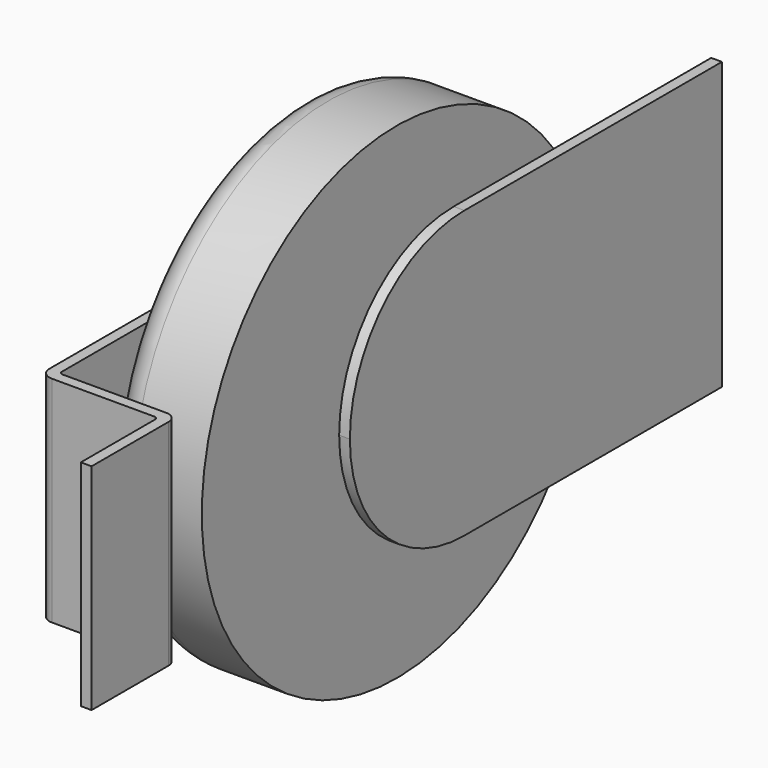
from build123d import *

# Parameters (mm, degrees)
F1_DEPTH      = 1.5
F1_DEPTH_BACK = 1.5
F4_DEPTH      = 2
F4_DEPTH_BACK = 2
F5_R          = 1.99999


# Not quite as in the source:
# - a fillet or chamfer is up to 0.001 mm smaller than in the source, because OpenCascade refuses the exact size


with BuildPart() as f1:
    # F0 (on Top) → F1 (new body, two sides)
    with BuildSketch(Plane.XY) as f1_sk:
        with BuildLine():
            Line((0.15, 1.5), (0, 1.5))
            Line((0, 1.5), (0, 0))
            Line((0, 0), (0, -4))
            ThreePointArc((0, -4), (0.0487994019, -4.1178121778), (0.1666115796, -4.1666115796))
            Line((0.1666115796, -4.1666115796), (1.6031347549, -4.1666115796))
            ThreePointArc((1.6031347549, -4.1666115796), (1.6362734875, -4.1803380921), (1.65, -4.2134768248))
            Line((1.65, -4.2134768248), (1.65, -5.5134768248))
            Line((1.65, -5.5134768248), (1.8, -5.5134768248))
            Line((1.8, -5.5134768248), (1.8, -4.1666115796))
            ThreePointArc((1.8, -4.1666115796), (1.7560660172, -4.0605455625), (1.65, -4.0166115796))
            Line((1.65, -4.0166115796), (0.1968652451, -4.0166115796))
            ThreePointArc((0.1968652451, -4.0166115796), (0.1637265125, -4.0028850671), (0.15, -3.9697463345))
            Line((0.15, -3.9697463345), (0.15, 0))
            Line((0.15, 0), (0.15, 1.5))
        make_face()
    extrude(amount=F1_DEPTH)
    extrude(f1_sk.sketch, amount=-F1_DEPTH_BACK)

    # F0 (on Top) → F2 (revolve)
    with BuildSketch(Plane.XY):
        with BuildLine():
            Line((0.15, 2.6), (0.15, 1.5))
            Line((0.15, 1.5), (0.15, 0))
            Line((0.15, 0), (0.3, 0))
            Line((0.3, 0), (0.3, 2.7))
            Line((0.3, 2.7), (0.25, 2.7))
            ThreePointArc((0.25, 2.7), (0.1792893219, 2.6707106781), (0.15, 2.6))
        make_face()
    revolve(axis=Axis((0.225, 0, 0), (-1, 0, 0)))

    # F0 (on Top) → F3 (revolve)
    with BuildSketch(Plane.XY):
        with BuildLine():
            Line((0.3, 2.7), (0.3, 0))
            Line((0.3, 0), (1.65, 0))
            Line((1.65, 0), (1.65, 3.4))
            Line((1.65, 3.4), (0.7, 3.4))
            ThreePointArc((0.7, 3.4), (0.4171572875, 3.2828427125), (0.3, 3))
            Line((0.3, 3), (0.3, 2.7))
        make_face()
    revolve(axis=Axis((0.975, 0, 0), (-1, 0, 0)))

    # F0 (on Top) → F4 (join, two sides)
    with BuildSketch(Plane.XY) as f4_sk:
        Polygon((1.65, 3.4), (1.65, 0), (1.65, -1), (1.8, -1), (1.8, 5.5), (1.65, 5.5), align=None)
    extrude(amount=F4_DEPTH)
    extrude(f4_sk.sketch, amount=-F4_DEPTH_BACK)

    # F5 (radius 2 in the source; OpenCascade refuses exactly that, so slightly less here)
    f5_edges = [f1.edges().sort_by_distance(p)[0] for p in [
        (1.725, -1, -2),
        (1.725, -1, 2),
    ]]
    fillet(f5_edges, radius=F5_R)


solid = f1.part
